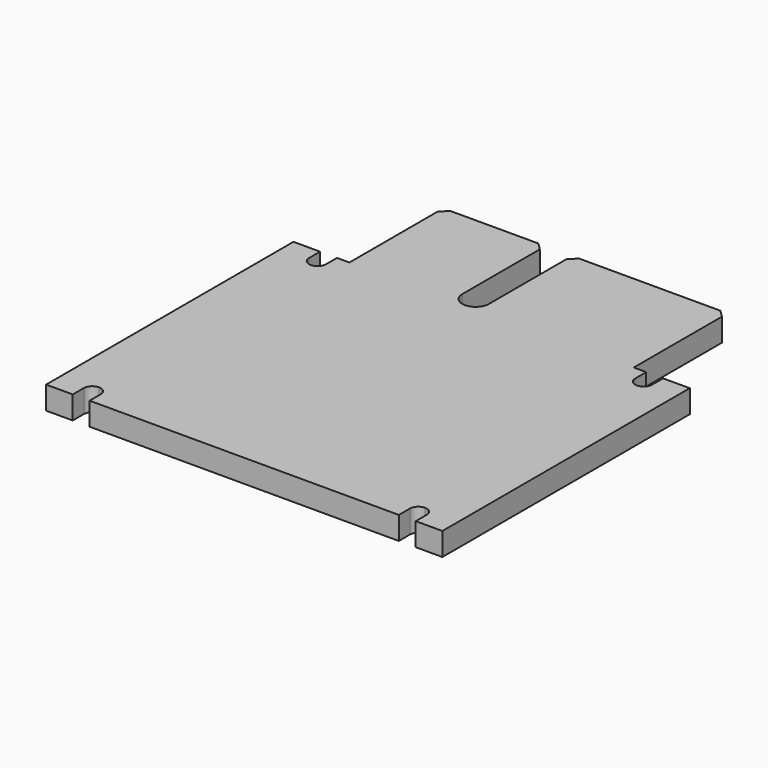
from build123d import *

# Parameters (mm, degrees)
F0_W     = 28.321
F0_H     = 30.48
F1_DEPTH = 1.64
F2_W     = 1.905
F2_H     = 8.382
F2_W_2   = 1.207
F2_H_2   = 1.5875
F3_DEPTH = 25
F4_R     = 0.95249
F5_SIZE  = 0.507
F6_R     = 0.60349


# Not quite as in the source:
# - a fillet or chamfer is up to 0.001 mm smaller than in the source, because OpenCascade refuses the exact size


with BuildPart() as f1:
    # F0 (on Top) → F1 (new body)
    with BuildSketch(Plane.XY):
        with Locations((0, -15.24)):
            Rectangle(F0_W, F0_H)
    extrude(amount=F1_DEPTH)

    # F2 (on Top) → F3 (cut)
    with BuildSketch(Plane.XY):
        Polygon((-10.1605, 0), (-14.1605, 0), (-14.1605, -8.382), (-12.2555, -8.382), (-12.2555, -9.9695), (-11.0485, -9.9695), (-11.0485, -8.382), (-10.1605, -8.382), align=None)
        with Locations((-1.905, -4.191)):
            Rectangle(F2_W, F2_H)
        Polygon((14.1605, -8.382), (14.1605, 0), (10.1595, 0), (10.1595, -8.382), (11.0485, -8.382), (11.0485, -9.9695), (12.2555, -9.9695), (12.2555, -8.382), align=None)
        with Locations((-11.652, -29.68625)):
            Rectangle(F2_W_2, F2_H_2)
        with Locations((11.652, -29.68625)):
            Rectangle(F2_W_2, F2_H_2)
    extrude(amount=F3_DEPTH, mode=Mode.SUBTRACT)

    # F4 (radius 0.9525 in the source; OpenCascade refuses exactly that, so slightly less here)
    f4_edges = [f1.edges().sort_by_distance(p)[0] for p in [
        (-2.8575, -8.382, 0.82),
        (-0.9525, -8.382, 0.82),
    ]]
    fillet(f4_edges, radius=F4_R)

    # F5
    f5_edges = [f1.edges().sort_by_distance(p)[0] for p in [
        (10.1595, 0, 0.82),
        (-0.9525, 0, 0.82),
        (-2.8575, 0, 0.82),
        (-10.1605, 0, 0.82),
    ]]
    chamfer(f5_edges, length=F5_SIZE)

    # F6 (radius 0.6035 in the source; OpenCascade refuses exactly that, so slightly less here)
    f6_edges = [f1.edges().sort_by_distance(p)[0] for p in [
        (12.2555, -28.8925, 0.82),
        (-12.2555, -28.8925, 0.82),
        (-11.0485, -28.8925, 0.82),
        (11.0485, -28.8925, 0.82),
        (11.0485, -9.9695, 0.82),
        (12.2555, -9.9695, 0.82),
        (-12.2555, -9.9695, 0.82),
        (-11.0485, -9.9695, 0.82),
    ]]
    fillet(f6_edges, radius=F6_R)


solid = f1.part
